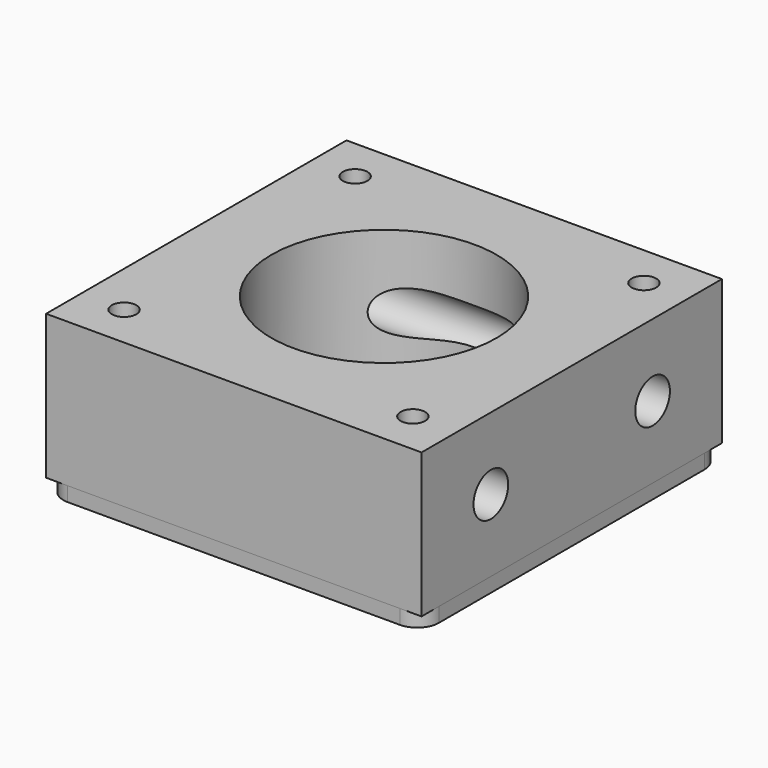
from build123d import *

# Parameters (mm, degrees)
F0_W     = 26
F0_H     = 26
F0_R     = 0.85
F0_R_2   = 7.8
F1_DEPTH = 10
F2_R     = 1.5
F3_DEPTH = 26.001
F4_R     = 0.85
F4_R_2   = 7.8
F4_R_3   = 1.5
F5_DEPTH = 1


with BuildPart() as f1:
    # F0 (on Top) → F1 (new body)
    with BuildSketch(Plane.XY):
        Rectangle(F0_W, F0_H)
        with Locations((-10, -10)):
            Circle(F0_R, mode=Mode.SUBTRACT)
        with Locations((10, -10)):
            Circle(F0_R, mode=Mode.SUBTRACT)
        with Locations((-10, 10)):
            Circle(F0_R, mode=Mode.SUBTRACT)
        Circle(F0_R_2, mode=Mode.SUBTRACT)
        with Locations((10, 10)):
            Circle(F0_R, mode=Mode.SUBTRACT)
    extrude(amount=F1_DEPTH)

    # F2 (on face) → F3 (cut, through all)
    with BuildSketch(Plane(origin=(-13, 0, 0), x_dir=(0, -1, 0), z_dir=(-1, 0, 0))):
        with Locations((-7, 5)):
            Circle(F2_R)
        with Locations((7, 5)):
            Circle(F2_R)
    extrude(amount=-F3_DEPTH, mode=Mode.SUBTRACT)


with BuildPart() as f5:
    # F4 (on face) → F5 (new body)
    with BuildSketch(Plane(origin=(0, 0, 0), x_dir=(1, 0, 0), z_dir=(0, 0, -1))):
        with BuildLine():
            ThreePointArc((-11.5, 13), (-12.5606601718, 12.5606601718), (-13, 11.5))
            Line((-13, 11.5), (-13, -11.5))
            ThreePointArc((-13, -11.5), (-12.5606601718, -12.5606601718), (-11.5, -13))
            Line((-11.5, -13), (11.5, -13))
            ThreePointArc((11.5, -13), (12.5606601718, -12.5606601718), (13, -11.5))
            Line((13, -11.5), (13, 11.5))
            ThreePointArc((13, 11.5), (12.5606601718, 12.5606601718), (11.5, 13))
            Line((11.5, 13), (-11.5, 13))
        make_face()
        with Locations((-10, -10)):
            Circle(F4_R, mode=Mode.SUBTRACT)
        with Locations((10, -10)):
            Circle(F4_R, mode=Mode.SUBTRACT)
        with Locations((-10, 10)):
            Circle(F4_R, mode=Mode.SUBTRACT)
        Circle(F4_R_2, mode=Mode.SUBTRACT)
        with Locations((10, 10)):
            Circle(F4_R, mode=Mode.SUBTRACT)
        Circle(F4_R_2)
        Circle(F4_R_3, mode=Mode.SUBTRACT)
    extrude(amount=F5_DEPTH)


solid = Compound([f1.part, f5.part])
